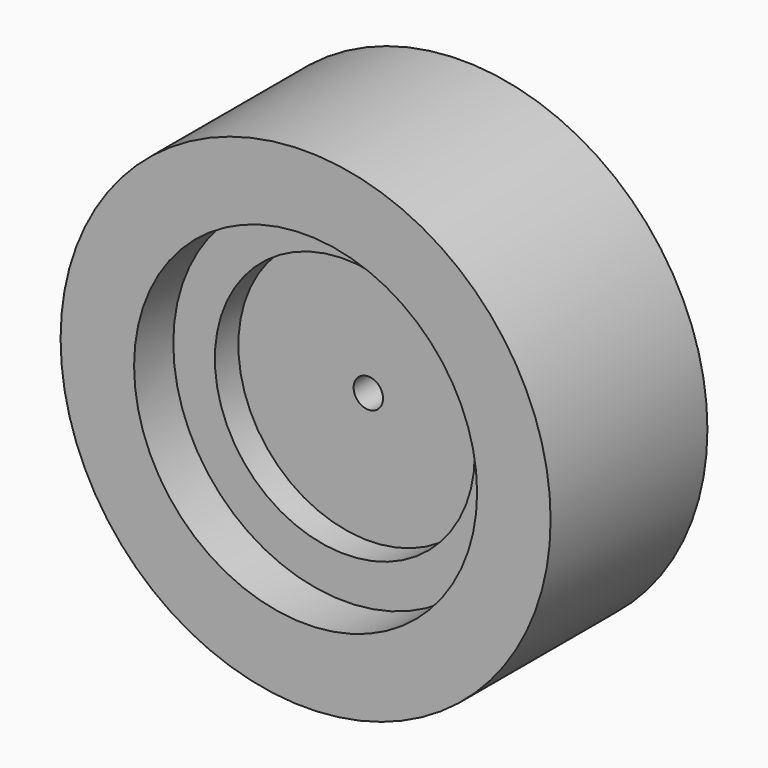
from build123d import *

# Parameters (mm, degrees)
F0_R     = 22.225
F0_R_2   = 16.8413804611
F1_DEPTH = 19.05
F0_R_3   = 31.75
F2_DEPTH = 25.4
F0_R_4   = 1.905
F4_DEPTH = 15.24


# Not quite as in the source:
# - the program builds the solid bodies; features that only make, move or delete a surface that nothing else refers to are left out


with BuildPart() as f1:
    # F0 (on Front) → F1 (new body)
    with BuildSketch(Plane.XZ):
        Circle(F0_R)
        Circle(F0_R_2, mode=Mode.SUBTRACT)
    extrude(amount=F1_DEPTH)

    # F0 (on Front) → F2 (join)
    with BuildSketch(Plane.XZ):
        Circle(F0_R_3)
        Circle(F0_R, mode=Mode.SUBTRACT)
    extrude(amount=F2_DEPTH)

    # F0 (on Front) → F4 (join)
    with BuildSketch(Plane.XZ):
        Circle(F0_R_2)
        Circle(F0_R_4, mode=Mode.SUBTRACT)
    extrude(amount=F4_DEPTH)


solid = f1.part
